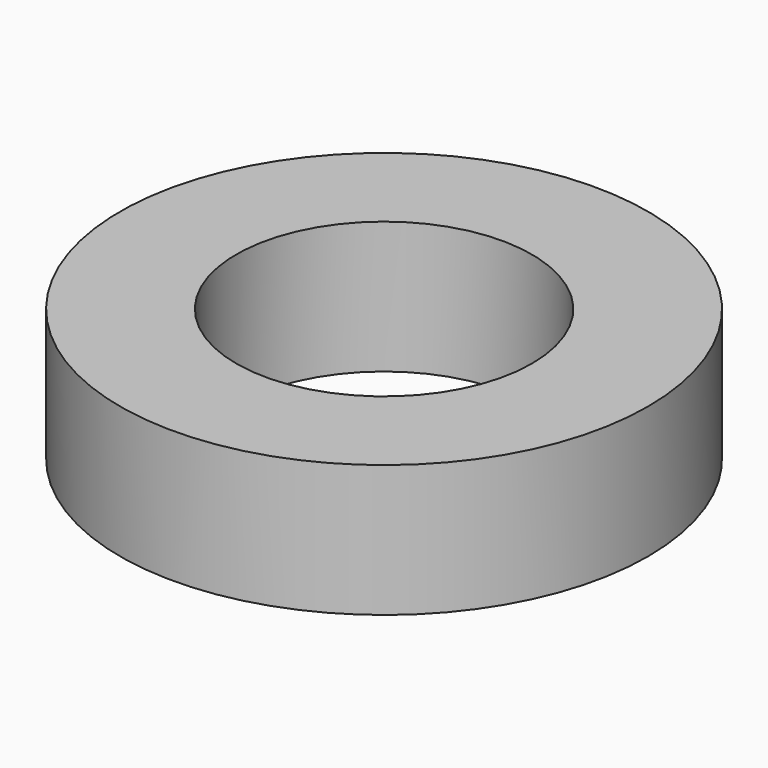
from build123d import *

# Parameters (mm, degrees)
F0_R     = 3.175
F0_R_2   = 1.778
F1_DEPTH = 1.5875


# Not quite as in the source:
# - a length typed as a fraction of an inch, garbled in the dataset ("3 / 203.2 mm" for 3/8 in), is restored


with BuildPart() as f1:
    # F0 (on Top) → F1 (new body)
    with BuildSketch(Plane.XY):
        Circle(F0_R)
        Circle(F0_R_2, mode=Mode.SUBTRACT)
    extrude(amount=F1_DEPTH)


solid = f1.part
